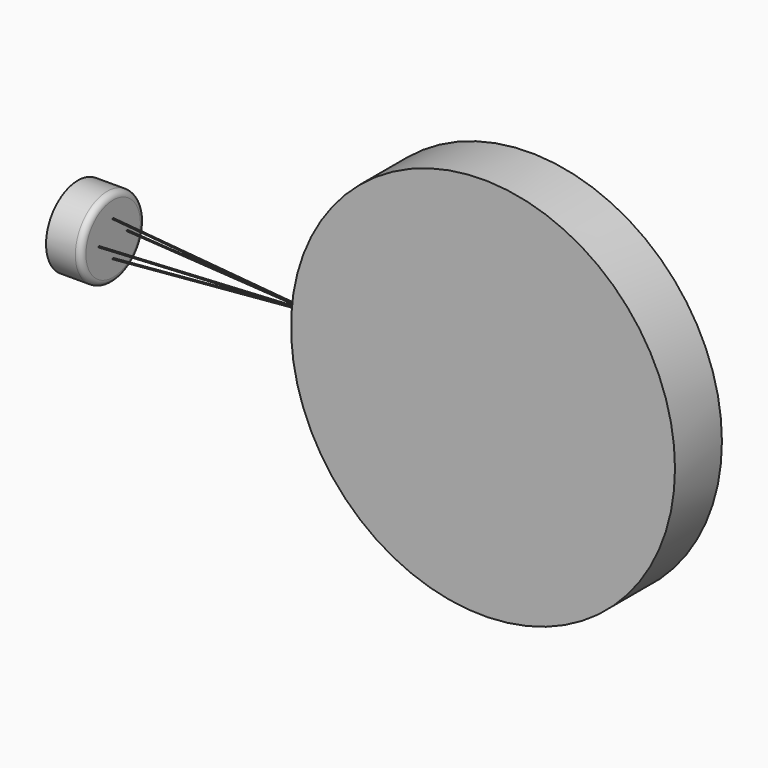
from build123d import *

# Parameters (mm, degrees)
F0_R           = 0.5
F5_COUNT       = 4
F1_R           = 34
F6_DEPTH       = 10
F7_R           = 4.99999
F9_R           = 34
F10_DEPTH      = 25
F11_R          = 163.6726572253
F12_DEPTH      = 25
F12_DEPTH_BACK = 25


# Not quite as in the source:
# - a fillet or chamfer is up to 0.001 mm smaller than in the source, because OpenCascade refuses the exact size


with BuildPart() as f3:
    # F3: sweep along a path in F2
    with BuildLine(Plane.XZ) as f3_path:
        Line((0, 15), (250, -6.8721658815))
    # F0 (on Right) → F3 (sweep)
    with BuildSketch(Plane.YZ):
        with Locations((0, 15)):
            Circle(F0_R)
    sweep(path=f3_path.line)


with BuildPart() as f5_1:
    # F5: instance of F3
    add(f3.part.rotate(Axis((150, 0, 0), (1, 0, 0)), 1 * 360 / F5_COUNT))


with BuildPart() as f5_2:
    # F5: instance of F3
    add(f3.part.rotate(Axis((150, 0, 0), (1, 0, 0)), 2 * 360 / F5_COUNT))


with BuildPart() as f5_3:
    # F5: instance of F3
    add(f3.part.rotate(Axis((150, 0, 0), (1, 0, 0)), 3 * 360 / F5_COUNT))


with BuildPart() as f6:
    # F1 (on Right) → F6 (new body)
    with BuildSketch(Plane.YZ):
        Circle(F1_R)
    extrude(amount=-F6_DEPTH)

    # F7 (radius 5 in the source; OpenCascade refuses exactly that, so slightly less here)
    f7_edges = [f6.edges().sort_by_distance(p)[0] for p in [
        (0, -34, 0),
        (-10, -34, 0),
    ]]
    fillet(f7_edges, radius=F7_R)


with BuildPart() as f10:
    # F9 (on offset) → F10 (new body)
    with BuildSketch(Plane.YZ.offset(-5)):
        Circle(F9_R)
    extrude(amount=-F10_DEPTH)


with BuildPart() as f12:
    # F11 (on Front) → F12 (new body, two sides)
    with BuildSketch(Plane.XZ) as f12_sk:
        with Locations((335.3325128555, 0)):
            Circle(F11_R)
    extrude(amount=F12_DEPTH)
    extrude(f12_sk.sketch, amount=-F12_DEPTH_BACK)


solid = Compound([f3.part, f5_1.part, f5_2.part, f5_3.part, f6.part, f10.part, f12.part])
